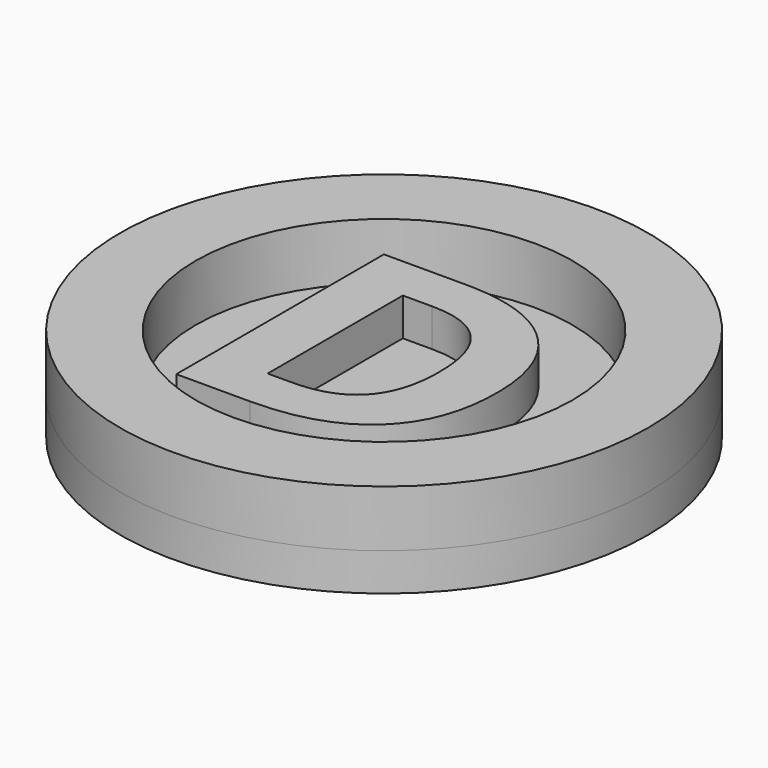
from build123d import *

# Parameters (mm, degrees)
F0_R         = 7
F0_R_2       = 5
F0_TEXT_SIZE = 9.638332879
F1_DEPTH     = 1
F2_DEPTH     = 1.5
F3_DEPTH     = 1


# Not quite as in the source:
# - Text() gives the source's letters only with a copy of the font that has no kerning and outlines rounded to 1/6400 em; it was checked with that copy


with BuildPart() as f1:
    # F0 (on Top) → F1 (new body)
    with BuildSketch(Plane.XY):
        Circle(F0_R)
        Circle(F0_R_2, mode=Mode.SUBTRACT)
        Circle(F0_R_2)
        with BuildLine():
            add(Edge.make_bspline(
                [(2.0428747735, 2.5217794384), (2.9750822816, 1.6324926314), (2.9750822816, 0.0361437483)],
                knots=[0, 0, 0, 1, 1, 1], degree=2))
            add(Edge.make_bspline(
                [(2.9750822816, 0.0361437483), (2.9750822816, -1.6626124216), (2.0074840199, -2.566206129)],
                knots=[0, 0, 0, 1, 1, 1], degree=2))
            add(Edge.make_bspline(
                [(2.0074840199, -2.566206129), (1.0398857583, -3.4697998364), (-0.7853735307, -3.4697998364)],
                knots=[0, 0, 0, 1, 1, 1], degree=2))
            Line((-0.7853735307, -3.4697998364), (-2.7341239596, -3.4697998364))
            Line((-2.7341239596, -3.4697998364), (-2.7341239596, 3.4110662454))
            Line((-2.7341239596, 3.4110662454), (-0.574534999, 3.4110662454))
            add(Edge.make_bspline(
                [(-0.574534999, 3.4110662454), (1.1106672653, 3.4110662454), (2.0428747735, 2.5217794384)],
                knots=[0, 0, 0, 1, 1, 1], degree=2))
        make_face(mode=Mode.SUBTRACT)
        with Locations((-3.6000679292, -3.4697998364)):
            Text('D', F0_TEXT_SIZE, font='Open Sans', font_style=FontStyle.BOLD, text_align=(TextAlign.LEFT, TextAlign.BOTTOM))
        with BuildLine():
            add(Edge.make_bspline(
                [(-0.6498344746, -2.2650082266), (1.4585508427, -2.2650082266), (1.4585508427, -0.0015059895)],
                knots=[0, 0, 0, 1, 1, 1], degree=2))
            add(Edge.make_bspline(
                [(1.4585508427, -0.0015059895), (1.4585508427, 2.2153105726), (-0.4992355233, 2.2153105726)],
                knots=[0, 0, 0, 1, 1, 1], degree=2))
            Line((-0.4992355233, 2.2153105726), (-1.2748201222, 2.2153105726))
            Line((-1.2748201222, 2.2153105726), (-1.2748201222, -2.2650082266))
            Line((-1.2748201222, -2.2650082266), (-0.6498344746, -2.2650082266))
        make_face()
    extrude(amount=-F1_DEPTH)


with BuildPart() as f2:
    # F0 (on Top) → F2 (new body)
    with BuildSketch(Plane.XY):
        Circle(F0_R)
        Circle(F0_R_2, mode=Mode.SUBTRACT)
    extrude(amount=F2_DEPTH)


with BuildPart() as f3:
    # F0 (on Top) → F3 (new body)
    with BuildSketch(Plane.XY):
        with Locations((-3.6000679292, -3.4697998364)):
            Text('D', F0_TEXT_SIZE, font='Open Sans', font_style=FontStyle.BOLD, text_align=(TextAlign.LEFT, TextAlign.BOTTOM))
    extrude(amount=F3_DEPTH)


solid = Compound([f1.part, f2.part, f3.part])
